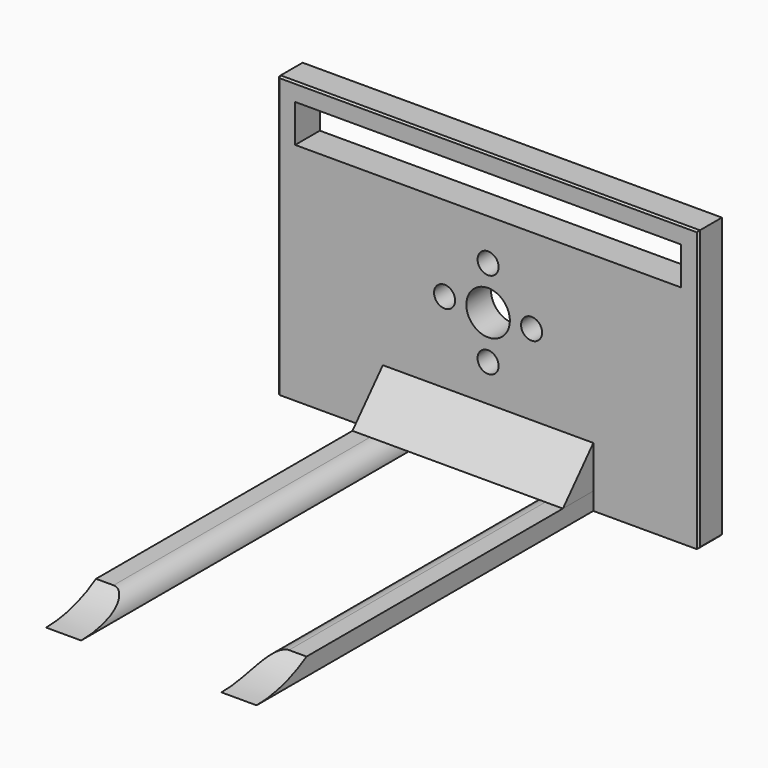
from build123d import *

# Parameters (mm, degrees)
F0_W      = 76.2
F0_H      = 50.8
F1_DEPTH  = 5.588
F2_W      = 6.35
F2_H      = 76.2
F3_DEPTH  = 3.175
F5_DEPTH  = 38.1
F6_W      = 47.7035964723
F6_H      = 3.175
F7_DEPTH  = 254
F8_R      = 3.937
F8_R_2    = 1.905
F9_DEPTH  = 25.4
F10_W     = 69.2231629074
F10_H     = 6.8492060885
F10_W_2   = 0.6268370926
F11_DEPTH = 25.4
F13_DEPTH = 254
F14_R     = 3.17499
F15_SIZE  = 0.3048


# Not quite as in the source:
# - a fillet or chamfer is up to 0.001 mm smaller than in the source, because OpenCascade refuses the exact size


with BuildPart() as f1:
    # F0 (on Front) → F1 (new body)
    with BuildSketch(Plane.XZ):
        Rectangle(F0_W, F0_H)
    extrude(amount=F1_DEPTH)

    # F2 (on face) → F3 (join)
    with BuildSketch(Plane(origin=(0, 0, -25.4), x_dir=(1, 0, 0), z_dir=(0, 0, -1))):
        with Locations((-15.875, 43.688)):
            Rectangle(F2_W, F2_H)
        with Locations((15.875, 43.688)):
            Rectangle(F2_W, F2_H)
    extrude(amount=-F3_DEPTH)

    # F8 (on face) → F9 (cut)
    with BuildSketch(Plane(origin=(0, 0, 0), x_dir=(-1, 0, 0), z_dir=(0, 1, 0))):
        Circle(F8_R)
        with Locations((0, 7.874)):
            Circle(F8_R_2)
        with Locations((0, -7.874)):
            Circle(F8_R_2)
        with Locations((7.874, 0)):
            Circle(F8_R_2)
        with Locations((-7.874, 0)):
            Circle(F8_R_2)
    extrude(amount=-F9_DEPTH, mode=Mode.SUBTRACT)

    # F10 (on face) → F11 (cut)
    with BuildSketch(Plane(origin=(0, 0, 0), x_dir=(-1, 0, 0), z_dir=(0, 1, 0))):
        with Locations((-0.3134185463, 18.8003969558)):
            Rectangle(F10_W, F10_H)
        with Locations((34.6115814537, 18.8003969558)):
            Rectangle(F10_W_2, F10_H)
    extrude(amount=-F11_DEPTH, mode=Mode.SUBTRACT)

    # F12 (on face) → F13 (cut)
    with BuildSketch(Plane.YZ.offset(19.05)):
        with BuildLine():
            ThreePointArc((-81.788, -25.4), (-75.9161354287, -24.5911900097), (-70.4816058278, -22.225))
            Line((-70.4816058278, -22.225), (-81.788, -22.225))
            Line((-81.788, -22.225), (-81.788, -25.4))
        make_face()
    extrude(amount=-F13_DEPTH, mode=Mode.SUBTRACT)

    # F14 (radius 3.175 in the source; OpenCascade refuses exactly that, so slightly less here)
    f14_edges = [f1.edges().sort_by_distance(p)[0] for p in [
        (-12.7, -38.034803, -22.225),
        (12.7, -38.034803, -22.225),
    ]]
    fillet(f14_edges, radius=F14_R)

    # F15
    f15_edges = [f1.edges().sort_by_distance(p)[0] for p in [
        (-38.1, -2.794, 25.4),
        (0, -5.588, 25.4),
        (-38.1, -5.588, 0),
        (38.1, -5.588, 0),
        (0, 0, 25.4),
        (38.1, 0, 0),
        (-38.1, 0, 0),
        (-38.1, -2.794, -25.4),
        (38.1, -2.794, -25.4),
    ]]
    chamfer(f15_edges, length=F15_SIZE)


with BuildPart() as f5:
    # F4 (on face) → F5 (new body)
    with BuildSketch(Plane(origin=(-19.05, 0, 0), x_dir=(0, -1, 0), z_dir=(-1, 0, 0))):
        Polygon((5.588, -22.225), (5.588, -25.4), (81.788, -25.4), (81.788, -22.225), (12.4667482451, -22.225), align=None)
        Polygon((5.588, -14.562738128), (5.588, -22.225), (12.4667482451, -22.225), align=None)
    extrude(amount=-F5_DEPTH)

    # F6 (on face) → F7 (cut)
    with BuildSketch(Plane(origin=(-19.05, 0, 0), x_dir=(0, -1, 0), z_dir=(-1, 0, 0))):
        with BuildLine():
            ThreePointArc((61.4126552725, -25.4), (57.2639609503, -24.038009454), (53.2915964723, -22.225))
            Line((53.2915964723, -22.225), (53.2915964723, -25.4))
            Line((53.2915964723, -25.4), (61.4126552725, -25.4))
        make_face()
        with BuildLine():
            Line((81.788, -22.225), (53.2915964723, -22.225))
            ThreePointArc((53.2915964723, -22.225), (57.2639609503, -24.038009454), (61.4126552725, -25.4))
            Line((61.4126552725, -25.4), (81.788, -25.4))
            Line((81.788, -25.4), (81.788, -22.225))
        make_face()
        with Locations((29.4397982361, -23.8125)):
            Rectangle(F6_W, F6_H)
        with BuildLine():
            Line((81.788, -25.4), (61.4126552725, -25.4))
            ThreePointArc((61.4126552725, -25.4), (71.6003276362, -26.7408633781), (81.788, -25.4))
        make_face()
    extrude(amount=-F7_DEPTH, mode=Mode.SUBTRACT)


solid = Compound([f1.part, f5.part])
